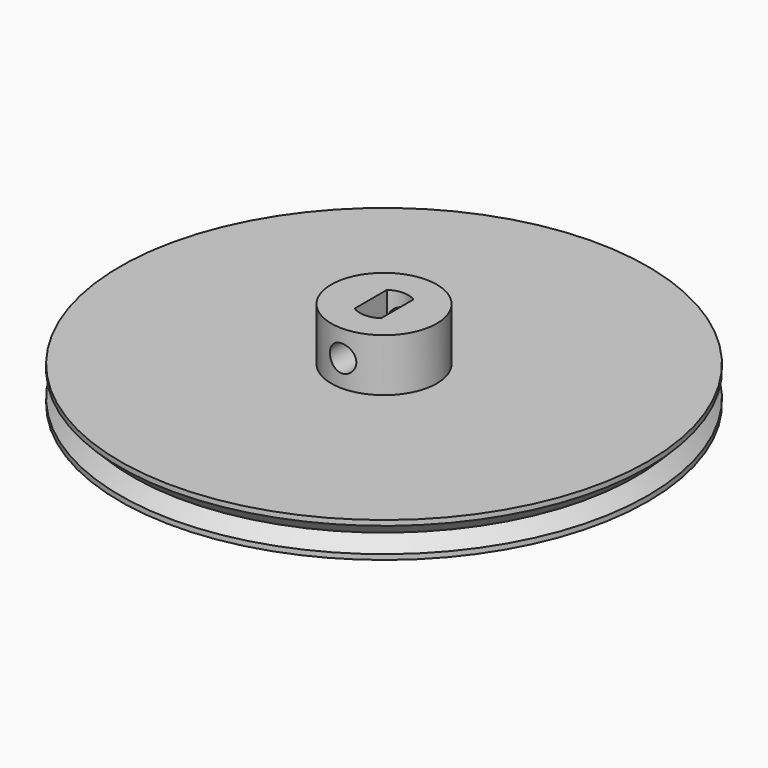
from build123d import *

# Parameters (mm, degrees)
F0_R     = 30
F0_R_2   = 6
F1_DEPTH = 4
F2_DEPTH = 6
F3_R     = 1.5
F4_DEPTH = 12.5
F5_W     = 3
F5_H     = 4.6
F6_DEPTH = 9.4


with BuildPart() as f1:
    # F0 (on Top) → F1 (new body)
    with BuildSketch(Plane.XY):
        Circle(F0_R)
        Circle(F0_R_2, mode=Mode.SUBTRACT)
        Circle(F0_R_2)
    extrude(amount=-F1_DEPTH)

    # F0 (on Top) → F2 (join)
    with BuildSketch(Plane.XY):
        Circle(F0_R_2)
    extrude(amount=F2_DEPTH)

    # F3 (on Front) → F4 (cut, symmetric)
    with BuildSketch(Plane.XZ):
        with Locations((0, 3)):
            Circle(F3_R)
    extrude(amount=F4_DEPTH, both=True, mode=Mode.SUBTRACT)

    # F5 (on face) → F6 (cut)
    with BuildSketch(Plane.XY.offset(6)):
        Rectangle(F5_W, F5_H)
        with BuildLine():
            Line((-1.5, 2.3), (1.5, 2.3))
            ThreePointArc((1.5, 2.3), (0, 2.7540939565), (-1.5, 2.3))
        make_face()
        with BuildLine():
            ThreePointArc((-1.5, -2.3), (0, -2.7459060435), (1.5, -2.3))
            Line((1.5, -2.3), (-1.5, -2.3))
        make_face()
    extrude(amount=-F6_DEPTH, mode=Mode.SUBTRACT)

    # F7 (on Front) → F8 (revolve, cut)
    with BuildSketch(Plane.XZ):
        Polygon((-28.5857864376, -2), (-30, -0.5857864376), (-30, -3.4142135624), align=None)
    revolve(axis=Axis((0, 0, 0.2672639675), (0, 0, -1)), mode=Mode.SUBTRACT)


solid = f1.part
